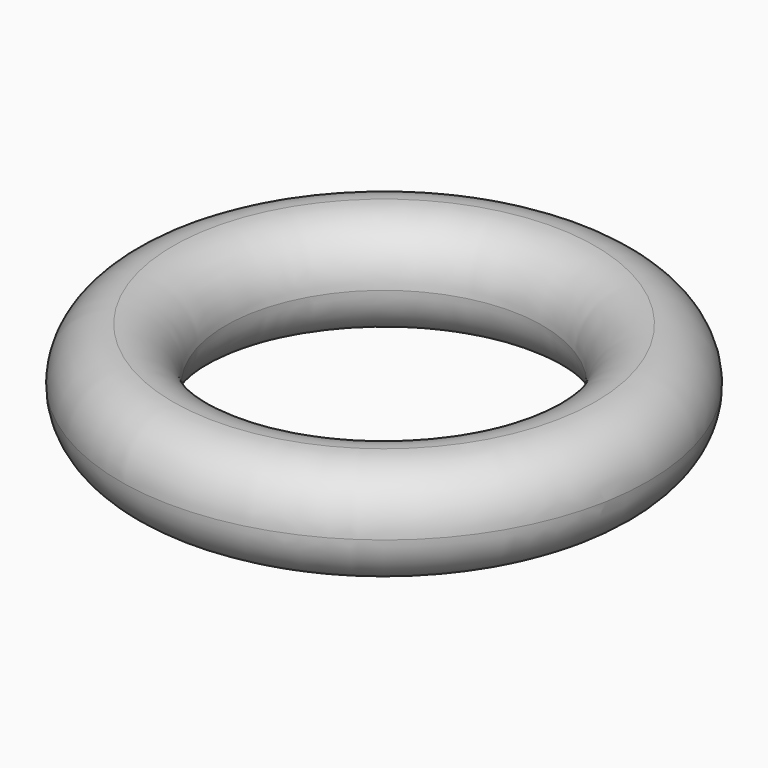
from build123d import *

# Parameters (mm, degrees)
F0_R     = 6.35
F0_R_2   = 3.81
F1_DEPTH = 2.54
F2_R     = 1.26999


# Not quite as in the source:
# - a fillet or chamfer is up to 0.001 mm smaller than in the source, because OpenCascade refuses the exact size


with BuildPart() as f1:
    # F0 (on Top) → F1 (new body)
    with BuildSketch(Plane.XY):
        Circle(F0_R)
        Circle(F0_R_2, mode=Mode.SUBTRACT)
    extrude(amount=F1_DEPTH)

    # F2 (radius 1.27 in the source; OpenCascade refuses exactly that, so slightly less here)
    f2_edges = [f1.edges().sort_by_distance(p)[0] for p in [
        (-6.35, 0, 2.54),
        (-6.35, 0, 0),
        (-3.81, 0, 2.54),
        (-3.81, 0, 0),
    ]]
    fillet(f2_edges, radius=F2_R)


solid = f1.part
